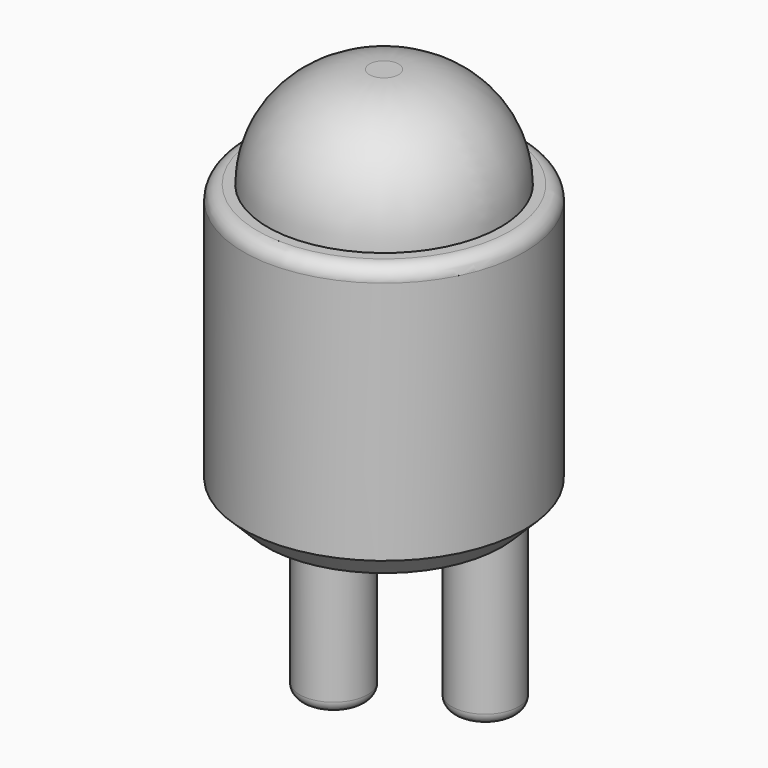
from build123d import *

# Parameters (mm, degrees)
F0_R          = 63.5
F1_DEPTH      = 63.5
F1_DEPTH_BACK = 63.5
F2_SIZE       = 10.16
F3_R          = 6.35
F4_R          = 52.5552622302
F5_DEPTH      = 45.72
F8_R          = 15.0932692433
F9_DEPTH      = 82.296
F10_R         = 5.08
F11_R         = 15.3989584518
F12_DEPTH     = 80.01
F13_R         = 5.08


# Not quite as in the source:
# - a fillet or chamfer that OpenCascade refuses, or shapes differently, is made with other operations: its cross-section is extruded or revolved along the edge and cut away or added


with BuildPart() as f1:
    # F0 (on Top) → F1 (new body, two sides)
    with BuildSketch(Plane.XY) as f1_sk:
        Circle(F0_R)
    extrude(amount=F1_DEPTH)
    extrude(f1_sk.sketch, amount=-F1_DEPTH_BACK)

    # F2
    f2_edges = [f1.edges().sort_by_distance(p)[0] for p in [
        (-63.5, 0, -63.5),
    ]]
    chamfer(f2_edges, length=F2_SIZE)

    # F3
    f3_edges = [f1.edges().sort_by_distance(p)[0] for p in [
        (-63.5, 0, 63.5),
    ]]
    fillet(f3_edges, radius=F3_R)

    # F4 (on face) → F5 (join)
    with BuildSketch(Plane.XY.offset(63.5)):
        Circle(F4_R)
    extrude(amount=F5_DEPTH)

    # F6: fillet of radius 45.9907683632 on 1 edges, made by hand


with BuildPart() as f6_tool2:
    # F6_s3 → F6_t4 (revolve)
    with BuildSketch(Plane.XZ):
        with BuildLine():
            ThreePointArc((52.5552622302, 63.2292316368), (39.0848780486, 95.7496158184), (6.564493867, 109.22))
            Line((6.564493867, 109.22), (52.5552622302, 109.22))
            Line((52.5552622302, 109.22), (52.5552622302, 63.2292316368))
        make_face()
    revolve(axis=Axis((0, 0, 109.22), (0, 0, 1)))

    split(bisect_by=Plane.XY.offset(63.5), keep=Keep.TOP)


with BuildPart() as f1_1:
    add(f1.part)

    # F6_t1: cut F6_tool2
    add(f6_tool2.part, mode=Mode.SUBTRACT)

    # F8 (on face) → F9 (join)
    with BuildSketch(Plane(origin=(0, 0, -63.5), x_dir=(1, 0, 0), z_dir=(0, 0, -1))):
        with Locations((26.5111289918, -24.0834727883)):
            Circle(F8_R)
    extrude(amount=F9_DEPTH)

    # F10
    f10_edges = [f1_1.edges().sort_by_distance(p)[0] for p in [
        (11.41786, 24.083473, -145.796),
    ]]
    fillet(f10_edges, radius=F10_R)

    # F11 (on face) → F12 (join)
    with BuildSketch(Plane(origin=(0, 0, -63.5), x_dir=(1, 0, 0), z_dir=(0, 0, -1))):
        with Locations((-18.4494890273, 5.414089188)):
            Circle(F11_R)
    extrude(amount=F12_DEPTH)

    # F13
    f13_edges = [f1_1.edges().sort_by_distance(p)[0] for p in [
        (-33.848447, -5.414089, -143.51),
    ]]
    fillet(f13_edges, radius=F13_R)


solid = f1_1.part
